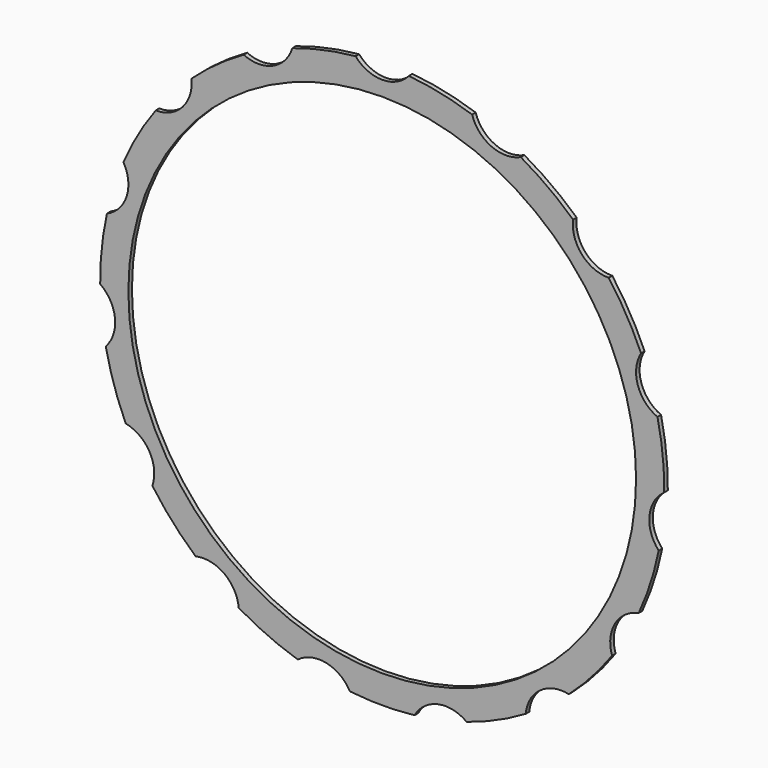
from build123d import *

# Parameters (mm, degrees)
F0_R            = 63.5
F0_R_2          = 57.15
F1_DEPTH        = 1
F3_DEPTH        = 12.7
F3_COPIES_COUNT = 15


# Not quite as in the source:
# - a pattern or mirror of a feature is missing from the dataset's text; its kind, count and spacing are read off the source's solid


with BuildPart() as f1:
    # F0 (on Front) → F1 (new body)
    with BuildSketch(Plane.XZ):
        Circle(F0_R)
        Circle(F0_R_2, mode=Mode.SUBTRACT)
    extrude(amount=F1_DEPTH)

    # F2 (on face) → F3 (cut, symmetric)
    with BuildSketch(Plane.XZ.offset(1)):
        with BuildLine():
            ThreePointArc((5.9974264065, 63.2161441129), (0, 63.5), (-5.9974264065, 63.2161441129))
            ThreePointArc((-5.9974264065, 63.2161441129), (0, 60.4966959565), (5.9974264065, 63.2161441129))
        make_face()
        with BuildLine():
            ThreePointArc((5.9974264065, 63.2161441129), (7.4628085396, 65.6633459283), (7.9730370433, 68.4697329998))
            ThreePointArc((7.9730370433, 68.4697329998), (-2.8063870715, 75.9325415394), (-5.9974264065, 63.2161441129))
            ThreePointArc((-5.9974264065, 63.2161441129), (0, 63.5), (5.9974264065, 63.2161441129))
        make_face()
    f3 = extrude(amount=F3_DEPTH, both=True, mode=Mode.SUBTRACT)

    # F3_copies: F3 ×15 about axis
    f3_copies_axis = Axis((0, 0, 0), (0, 1, 0))
    for i in range(1, F3_COPIES_COUNT):
        add(f3.rotate(f3_copies_axis, i * 360 / F3_COPIES_COUNT), mode=Mode.SUBTRACT)


solid = f1.part
